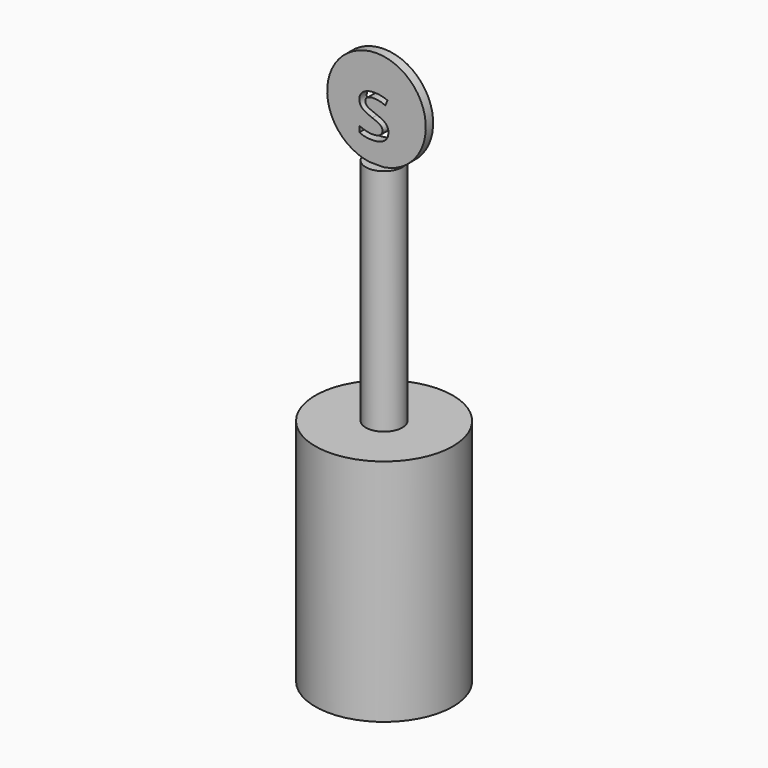
from build123d import *

# Parameters (mm, degrees)
F0_R         = 3.81
F1_DEPTH     = 12.7
F2_R         = 1.016
F3_DEPTH     = 25.4
F4_R         = 2.7319833643
F5_DEPTH     = 0.508
F6_TEXT_SIZE = 4.2397787588
F7_DEPTH     = 3.811


# Not quite as in the source:
# - Text() gives the source's letters only with a copy of the font that has no kerning and outlines rounded to 1/6400 em; it was checked with that copy


with BuildPart() as f1:
    # F0 (on Top) → F1 (new body)
    with BuildSketch(Plane.XY):
        Circle(F0_R)
    extrude(amount=F1_DEPTH)

    # F2 (on Top) → F3 (join)
    with BuildSketch(Plane.XY):
        Circle(F2_R)
    extrude(amount=F3_DEPTH)

    # F4 (on Front) → F5 (join)
    with BuildSketch(Plane.XZ):
        with Locations((-0.0132167179, 28.1032640487)):
            Circle(F4_R)
    extrude(amount=F5_DEPTH)

    # F6 (on Front) → F7 (cut, through all)
    with BuildSketch(Plane.XZ):
        with Locations((-1.1814190075, 26.5633612871)):
            Text('s', F6_TEXT_SIZE, font='Open Sans', text_align=(TextAlign.LEFT, TextAlign.BOTTOM))
    extrude(amount=F7_DEPTH, mode=Mode.SUBTRACT)


solid = f1.part
